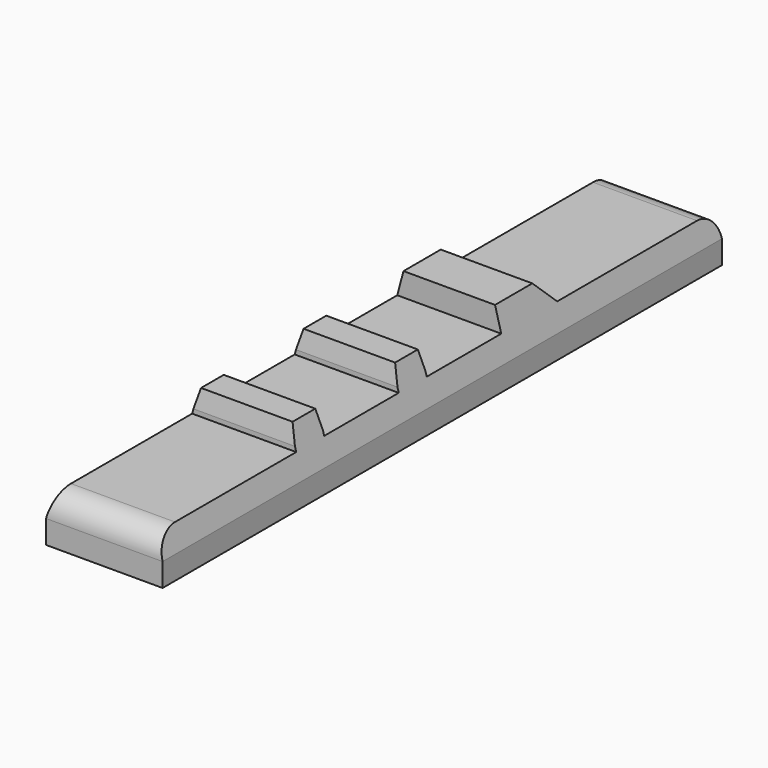
from build123d import *

# Parameters (mm, degrees)
F1_DEPTH    = 6.35
F2_SIZE2    = 0.1791482124
F2_SIZE     = 1.016
F2_2_SIZE2  = 0.1791482124
F2_2_SIZE   = 1.016
F2_3_SIZE2  = 0.1791482124
F2_3_SIZE   = 1.016
F3_SIZE2    = 0.1791482124
F3_SIZE     = 1.016
F4_SIZE2    = 0.6805909488
F4_SIZE     = 2.54
F5_SIZE2    = 0.6805909488
F5_SIZE     = 2.54
F6_T4_DEPTH = 18.0529676813


# Not quite as in the source:
# - a fillet or chamfer that OpenCascade refuses, or shapes differently, is made with other operations: its cross-section is extruded or revolved along the edge and cut away or added


with BuildPart() as f1:
    # F0 (on Right) → F1 (new body)
    with BuildSketch(Plane.YZ):
        with BuildLine():
            Line((0, 1.27), (0, 0))
            Line((0, 0), (38.1, 0))
            Line((38.1, 0), (38.1, 1.27))
            ThreePointArc((38.1, 1.27), (37.7280256121, 2.1680256121), (36.83, 2.54))
            Line((36.83, 2.54), (28.575, 2.54))
            Line((28.575, 2.54), (28.575, 3.81))
            Line((28.575, 3.81), (23.495, 3.81))
            Line((23.495, 3.81), (23.495, 2.54))
            Line((23.495, 2.54), (18.415, 2.54))
            Line((18.415, 2.54), (18.415, 3.81))
            Line((18.415, 3.81), (16.51, 3.81))
            Line((16.51, 3.81), (16.51, 2.54))
            Line((16.51, 2.54), (11.43, 2.54))
            Line((11.43, 2.54), (11.43, 3.81))
            Line((11.43, 3.81), (9.525, 3.81))
            Line((9.525, 3.81), (9.525, 2.54))
            Line((9.525, 2.54), (1.27, 2.54))
            ThreePointArc((1.27, 2.54), (0.3719743879, 2.1680256121), (0, 1.27))
        make_face()
    extrude(amount=F1_DEPTH)

    # F2
    f2_edges = [f1.edges().sort_by_distance(p)[0] for p in [
        (3.175, 11.43, 3.81),
    ]]
    f2_side = f1.faces().sort_by_distance((3.175, 11.43, 3.175))[0]
    chamfer(f2_edges, length=F2_SIZE, length2=F2_SIZE2, reference=f2_side)

    # F2#2
    f2_2_edges = [f1.edges().sort_by_distance(p)[0] for p in [
        (3.175, 9.525, 3.81),
    ]]
    f2_2_side = f1.faces().sort_by_distance((3.175, 9.525, 3.175))[0]
    chamfer(f2_2_edges, length=F2_2_SIZE, length2=F2_2_SIZE2, reference=f2_2_side)

    # F2#3
    f2_3_edges = [f1.edges().sort_by_distance(p)[0] for p in [
        (3.175, 18.415, 3.81),
    ]]
    f2_3_side = f1.faces().sort_by_distance((3.175, 18.415, 3.175))[0]
    chamfer(f2_3_edges, length=F2_3_SIZE, length2=F2_3_SIZE2, reference=f2_3_side)

    # F3
    f3_edges = [f1.edges().sort_by_distance(p)[0] for p in [
        (3.175, 16.51, 3.81),
    ]]
    f3_side = f1.faces().sort_by_distance((3.175, 16.51, 3.175))[0]
    chamfer(f3_edges, length=F3_SIZE, length2=F3_SIZE2, reference=f3_side)

    # F4
    f4_edges = [f1.edges().sort_by_distance(p)[0] for p in [
        (6.35, 10.4775, 3.81),
    ]]
    f4_side = f1.faces().sort_by_distance((6.35, 19.258705, 1.457125))[0]
    chamfer(f4_edges, length=F4_SIZE, length2=F4_SIZE2, reference=f4_side)

    # F5
    f5_edges = [f1.edges().sort_by_distance(p)[0] for p in [
        (0, 17.4625, 3.81),
    ]]
    f5_side = f1.faces().sort_by_distance((0, 19.258705, 1.457125))[0]
    chamfer(f5_edges, length=F5_SIZE, length2=F5_SIZE2, reference=f5_side)

    # F6: chamfer of 2.54 on 1 edges, made by hand


with BuildPart() as f6_tool2:
    # F6_s3 → F6_t4 (new body)
    with BuildSketch(Plane.YZ.offset(-5.8514838407)):
        Polygon((28.575, 1.27), (26.035, 3.81), (28.575, 3.81), align=None)
    extrude(amount=F6_T4_DEPTH)

    split(bisect_by=Plane.XY.offset(2.54), keep=Keep.TOP)


with BuildPart() as f1_1:
    add(f1.part)

    # F6_t1: cut F6_tool2
    add(f6_tool2.part, mode=Mode.SUBTRACT)


solid = f1_1.part
